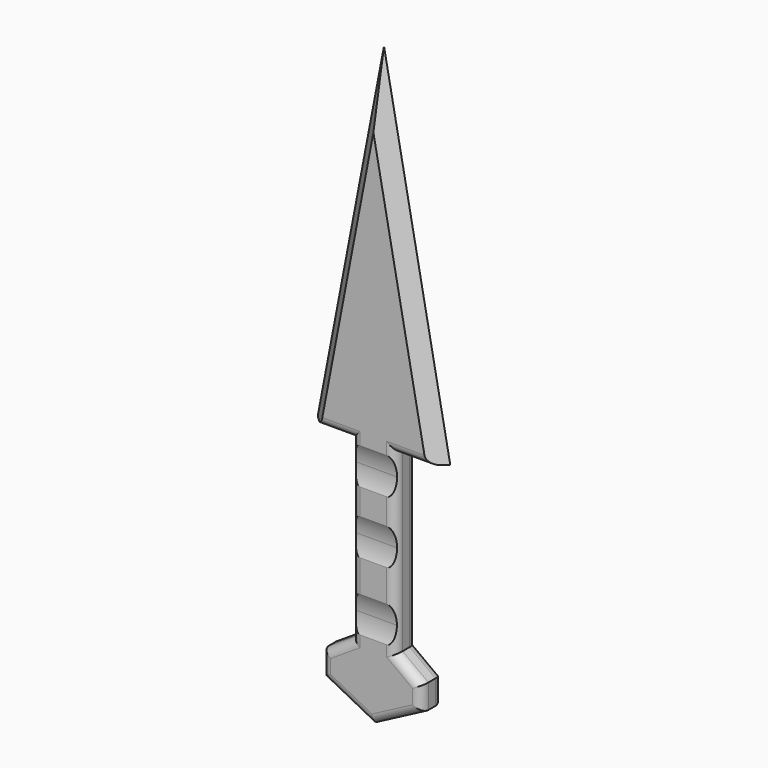
from build123d import *

# Parameters (mm, degrees)
F1_DEPTH = 3.81
F2_SIZE  = 1.90499
F3_R     = 1.27
F5_DEPTH = 25.4


# Not quite as in the source:
# - a fillet or chamfer is up to 0.001 mm smaller than in the source, because OpenCascade refuses the exact size
# - a feature names something its author has since deleted; it is built from what else it names


with BuildPart() as f1:
    # F0 (on Front) → F1 (new body)
    with BuildSketch(Plane.XZ):
        Polygon((-12.1744828463, 16.8822405368), (-12.1744828463, -8.5177594632), (-16.408668831, -11.2550966442), (-16.408668831, -14.7449430078), (-9.2011271045, -18.4709690511), (-2.1051054355, -14.7449430078), (-2.1051054355, -11.2550966442), (-5.8244828463, -8.5177594632), (-5.8244828463, 16.8822405368), (0.5255171537, 16.8822405368), (-8.9994828463, 66.7812823613), (-18.5244828463, 16.8822405368), align=None)
    extrude(amount=F1_DEPTH)

    # F2 (size 1.905 in the source; OpenCascade refuses exactly that, so slightly less here)
    f2_edges = [f1.edges().sort_by_distance(p)[0] for p in [
        (-13.761983, -3.81, 41.831761),
        (-4.236983, -3.81, 41.831761),
        (-13.761983, 0, 41.831761),
        (-4.236983, 0, 41.831761),
    ]]
    chamfer(f2_edges, length=F2_SIZE)

    # F3
    f3_edges = [f1.edges().sort_by_distance(p)[0] for p in [
        (-12.174483, -3.81, 4.182241),
        (-5.824483, -3.81, 4.182241),
        (-12.174483, 0, 4.182241),
        (-5.824483, 0, 4.182241),
        (-14.37979, -3.81, 16.882241),
        (-3.619176, 0, 16.882241),
        (-3.619176, -3.81, 16.882241),
        (-14.37979, 0, 16.882241),
        (-14.291576, -3.81, -9.886428),
        (-16.408669, -3.81, -13.00002),
        (-12.804898, -3.81, -16.607956),
        (-5.653116, -3.81, -16.607956),
        (-2.105105, -3.81, -13.00002),
        (-3.964794, -3.81, -9.886428),
        (-14.291576, 0, -9.886428),
        (-3.964794, 0, -9.886428),
        (-2.105105, 0, -13.00002),
        (-5.653116, 0, -16.607956),
        (-12.804898, 0, -16.607956),
        (-16.408669, 0, -13.00002),
    ]]
    fillet(f3_edges, radius=F3_R)

    # F4 (on Right) → F5 (cut)
    with BuildSketch(Plane.YZ):
        with BuildLine():
            ThreePointArc((-5.1016697734, 9.2693595216), (-3.730698506, 11.3268088009), (-3.2493867144, 13.7518858537))
            ThreePointArc((-3.2493867144, 13.7518858537), (-12.0244637672, 19.6205740621), (-14.0971036554, 9.2693595216))
            ThreePointArc((-14.0971036554, 9.2693595216), (-9.5993867144, 11.1368331894), (-5.1016697734, 9.2693595216))
        make_face()
        with BuildLine():
            ThreePointArc((-5.1016697734, 9.2693595216), (-9.5993867144, 11.1368331894), (-14.0971036554, 9.2693595216))
            ThreePointArc((-14.0971036554, 9.2693595216), (-9.5993867144, 7.4018858537), (-5.1016697734, 9.2693595216))
        make_face()
        with BuildLine():
            ThreePointArc((-5.1016697734, 9.2693595216), (-9.5993867144, 7.4018858537), (-14.0971036554, 9.2693595216))
            ThreePointArc((-14.0971036554, 9.2693595216), (-15.9420131796, 4.4809091421), (-13.6448170782, -0.107754962))
            ThreePointArc((-13.6448170782, -0.107754962), (-9.6056271037, 1.3330596991), (-5.571670106, -0.1223417843))
            ThreePointArc((-5.571670106, -0.1223417843), (-3.8592429678, 2.0714603295), (-3.2493867144, 4.7868331894))
            ThreePointArc((-3.2493867144, 4.7868331894), (-3.730698506, 7.2119102423), (-5.1016697734, 9.2693595216))
        make_face()
        with BuildLine():
            ThreePointArc((-5.571670106, -0.1223417843), (-9.6108600804, -1.5631564454), (-13.6448170782, -0.107754962))
            ThreePointArc((-13.6448170782, -0.107754962), (-12.3324733297, -10.7570736823), (-3.2671004698, -5.0169299357))
            ThreePointArc((-3.2671004698, -5.0169299357), (-3.8720598777, -2.311932968), (-5.571670106, -0.1223417843))
        make_face()
        with BuildLine():
            ThreePointArc((-5.571670106, -0.1223417843), (-9.6056271037, 1.3330596991), (-13.6448170782, -0.107754962))
            ThreePointArc((-13.6448170782, -0.107754962), (-9.6108600804, -1.5631564454), (-5.571670106, -0.1223417843))
        make_face()
    extrude(amount=-F5_DEPTH, mode=Mode.SUBTRACT)


solid = f1.part
